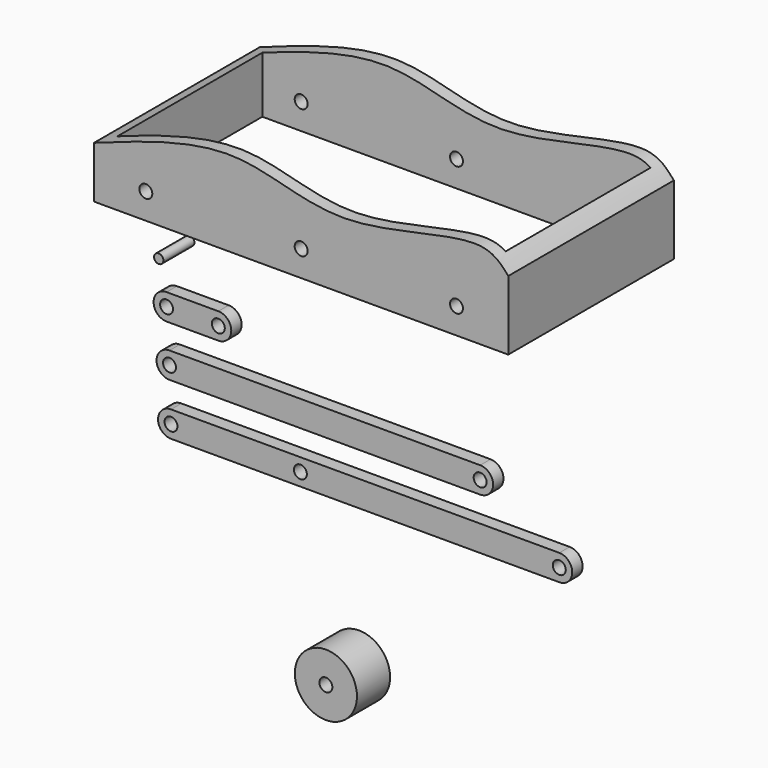
from build123d import *

# Parameters (mm, degrees)
F1_R      = 1.25
F2_DEPTH  = 2.5
F3_R      = 1.25
F4_DEPTH  = 2.5
F5_R      = 1.25
F6_DEPTH  = 2.5
F8_W      = 80
F8_H      = 40
F8_W_2    = 75
F8_H_2    = 35
F9_DEPTH  = 20
F10_R     = 1.25
F11_DEPTH = 40.001
F12_R     = 0.9
F13_DEPTH = 7.5
F15_DEPTH = 40.001
F16_R     = 6
F16_R_2   = 1.25
F17_DEPTH = 8


with BuildPart() as f2:
    # F1 (on Front) → F2 (new body)
    with BuildSketch(Plane.XZ):
        with BuildLine():
            Line((10, 2.5), (0, 2.5))
            ThreePointArc((0, 2.5), (-2.5, 0), (0, -2.5))
            Line((0, -2.5), (10, -2.5))
            ThreePointArc((10, -2.5), (12.5, 0), (10, 2.5))
        make_face()
        Circle(F1_R, mode=Mode.SUBTRACT)
        with Locations((10, 0)):
            Circle(F1_R, mode=Mode.SUBTRACT)
    extrude(amount=F2_DEPTH)


with BuildPart() as f4:
    # F3 (on Front) → F4 (new body)
    with BuildSketch(Plane.XZ):
        with BuildLine():
            Line((60.5706622079, -7.232673876), (0.5706622079, -7.232673876))
            ThreePointArc((0.5706622079, -7.232673876), (-1.9293377921, -9.732673876), (0.5706622079, -12.232673876))
            Line((0.5706622079, -12.232673876), (60.5706622079, -12.232673876))
            ThreePointArc((60.5706622079, -12.232673876), (63.0706622079, -9.732673876), (60.5706622079, -7.232673876))
        make_face()
        with Locations((0.5706622079, -9.732673876)):
            Circle(F3_R, mode=Mode.SUBTRACT)
        with Locations((60.5706622079, -9.732673876)):
            Circle(F3_R, mode=Mode.SUBTRACT)
    extrude(amount=F4_DEPTH)


with BuildPart() as f6:
    # F5 (on Front) → F6 (new body)
    with BuildSketch(Plane.XZ):
        with BuildLine():
            Line((75.8570737601, -17.1626018733), (0.8570737601, -17.1626018733))
            ThreePointArc((0.8570737601, -17.1626018733), (-1.6429262399, -19.6626018733), (0.8570737601, -22.1626018733))
            Line((0.8570737601, -22.1626018733), (75.8570737601, -22.1626018733))
            ThreePointArc((75.8570737601, -22.1626018733), (78.3570737601, -19.6626018733), (75.8570737601, -17.1626018733))
        make_face()
        with Locations((0.8570737601, -19.6626018733)):
            Circle(F5_R, mode=Mode.SUBTRACT)
        with Locations((25.8570737601, -19.6626018733)):
            Circle(F5_R, mode=Mode.SUBTRACT)
        with Locations((75.8570737601, -19.6626018733)):
            Circle(F5_R, mode=Mode.SUBTRACT)
    extrude(amount=F6_DEPTH)


with BuildPart() as f9:
    # F8 (on offset) → F9 (new body)
    with BuildSketch(Plane.XY.offset(25)):
        with Locations((40, 0)):
            Rectangle(F8_W, F8_H)
        with Locations((40, 0)):
            Rectangle(F8_W_2, F8_H_2, mode=Mode.SUBTRACT)
    extrude(amount=F9_DEPTH)

    # F10 (on face) → F11 (cut, through all)
    with BuildSketch(Plane.XZ.offset(20)):
        with Locations((10, 30)):
            Circle(F10_R)
        with Locations((70, 30)):
            Circle(F10_R)
        with Locations((40, 30)):
            Circle(F10_R)
    extrude(amount=-F11_DEPTH, mode=Mode.SUBTRACT)

    # F14 (on face) → F15 (cut, through all)
    with BuildSketch(Plane.XZ.offset(20)):
        with BuildLine():
            Line((-10.1319709793, 49.101550132), (0, 35))
            add(Edge.make_bspline(
                [(0, 35), (9.529848485, 38.4259781723), (27.4495666781, 44.8681124286), (47.1159441406, 34.1178456935), (74.6396223756, 44.5048404906), (78.6707572882, 39.8923398991), (80, 38.3713953197)],
                knots=[0, 0, 0, 0, 0.300472275, 0.5650014794, 0.8565618304, 1, 1, 1, 1], degree=3))
            Line((80, 38.3713953197), (95.8632975817, 42.5701513886))
            Line((95.8632975817, 42.5701513886), (68.1515038013, 61.1379854381))
            Line((68.1515038013, 61.1379854381), (-10.1319709793, 49.101550132))
        make_face()
    extrude(amount=-F15_DEPTH, mode=Mode.SUBTRACT)


with BuildPart() as f13:
    # F12 (on Front) → F13 (new body)
    with BuildSketch(Plane.XZ):
        with Locations((2.488047583, 11.0218990594)):
            Circle(F12_R)
    extrude(amount=F13_DEPTH)


with BuildPart() as f17:
    # F16 (on Front) → F17 (new body)
    with BuildSketch(Plane.XZ):
        with Locations((35.1786203682, -50.5970679224)):
            Circle(F16_R)
        with Locations((35.1786203682, -50.5970679224)):
            Circle(F16_R_2, mode=Mode.SUBTRACT)
    extrude(amount=F17_DEPTH)


solid = Compound([f2.part, f4.part, f6.part, f9.part, f13.part, f17.part])
